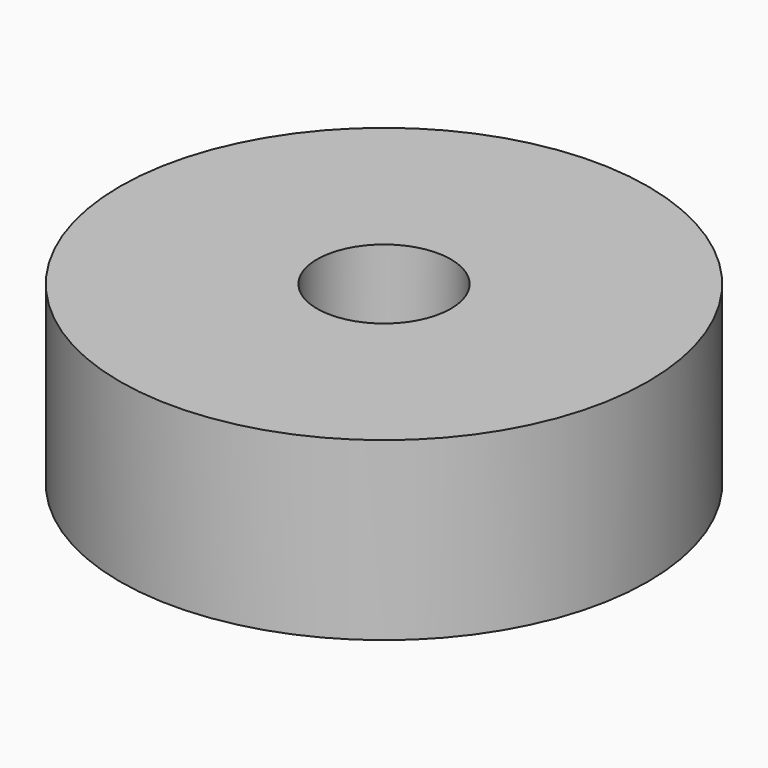
from build123d import *

# Parameters (mm, degrees)
F0_R     = 9.525
F0_R_2   = 2.413
F1_DEPTH = 6.35


# Not quite as in the source:
# - a length typed as a fraction of an inch, garbled in the dataset ("3 / 203.2 mm" for 3/8 in), is restored


with BuildPart() as f1:
    # F0 (on Top) → F1 (new body)
    with BuildSketch(Plane.XY):
        Circle(F0_R)
        Circle(F0_R_2, mode=Mode.SUBTRACT)
    extrude(amount=F1_DEPTH)


solid = f1.part
